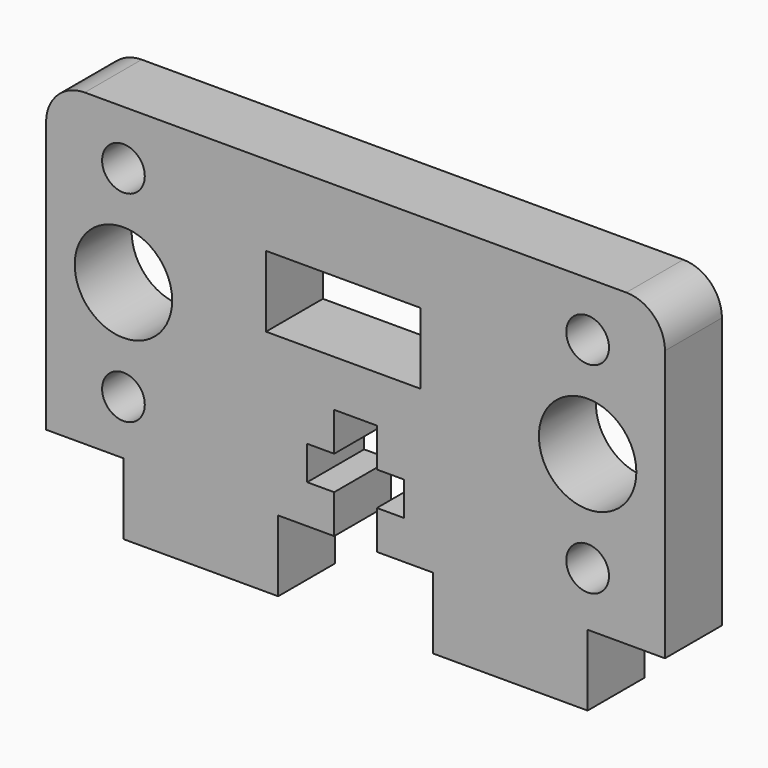
from build123d import *

# Parameters (mm, degrees)
F0_R     = 1.7526
F0_R_2   = 4
F0_W     = 12.7
F0_H     = 5.842
F1_DEPTH = 5.842
F2_R     = 3.175


# Not quite as in the source:
# - a feature names something its author has since deleted; it is built from what else it names


with BuildPart() as f1:
    # F0 (on Front) → F1 (new body)
    with BuildSketch(Plane.XZ):
        Polygon((-12.7, 12.7), (-25.4, 12.7), (-25.4, -12.7), (-19.05, -12.7), (-19.05, -18.542), (-6.35, -18.542), (-6.35, -12.7), (-1.7526, -12.7), (-1.7526, -9.525), (-3.96875, -9.525), (-3.96875, -6.746875), (-1.7526, -6.746875), (-1.7526, -3.571875), (1.7526, -3.571875), (1.7526, -6.746875), (3.96875, -6.746875), (3.96875, -9.525), (1.7526, -9.525), (1.7526, -12.7), (6.35, -12.7), (6.35, -18.542), (19.05, -18.542), (19.05, -12.7), (25.4, -12.7), (25.4, 12.7), (12.7, 12.7), align=None)
        with Locations((-19.05, -8.255)):
            Circle(F0_R, mode=Mode.SUBTRACT)
        with Locations((19.05, -8.255)):
            Circle(F0_R, mode=Mode.SUBTRACT)
        with Locations((-19.05, 0)):
            Circle(F0_R_2, mode=Mode.SUBTRACT)
        with Locations((-1, 3.175)):
            Rectangle(F0_W, F0_H, mode=Mode.SUBTRACT)
        with Locations((-19.05, 8.255)):
            Circle(F0_R, mode=Mode.SUBTRACT)
        with Locations((19.05, 0)):
            Circle(F0_R_2, mode=Mode.SUBTRACT)
        with Locations((19.05, 8.255)):
            Circle(F0_R, mode=Mode.SUBTRACT)
    extrude(amount=F1_DEPTH)

    # F2
    f2_edges = [f1.edges().sort_by_distance(p)[0] for p in [
        (-25.4, -2.921, 12.7),
        (25.4, -2.921, 12.7),
    ]]
    fillet(f2_edges, radius=F2_R)


solid = f1.part
